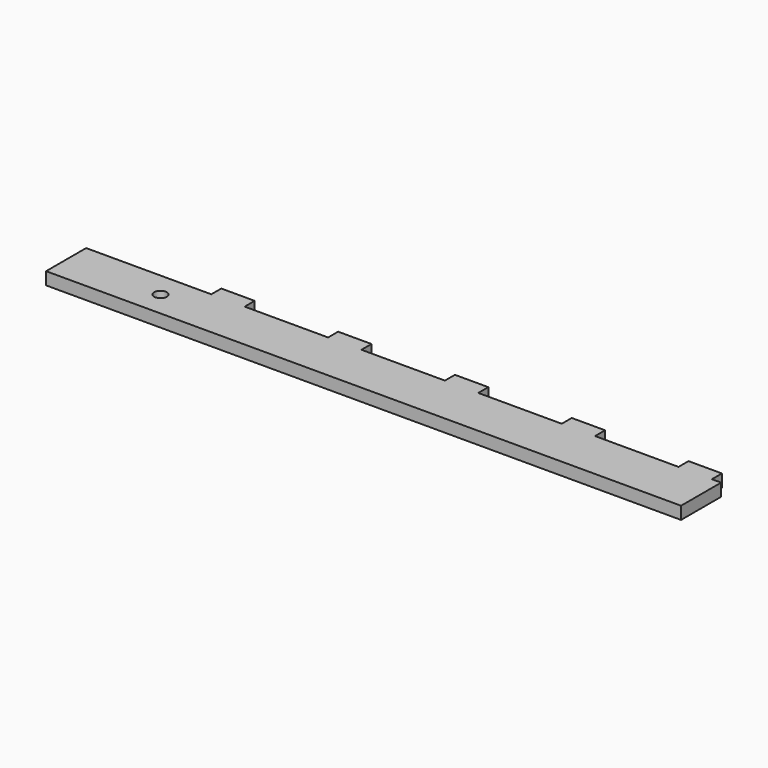
from build123d import *

# Parameters (mm, degrees)
F0_W     = 1143
F0_H     = 76.2
F1_DEPTH = 19.05
F2_W     = 50.8
F2_H     = 19.05
F3_DEPTH = 19.05
F4_R     = 9.525
F5_DEPTH = 19.05
F6_W     = 22.86
F6_H     = 15.875
F7_DEPTH = 25.4
F9_DEPTH = 25.4


# Not quite as in the source:
# - a length typed as a fraction of an inch, garbled in the dataset ("3 / 203.2 mm" for 3/8 in), is restored
# - a feature names something its author has since deleted; it is built from what else it names


with BuildPart() as f1:
    # F0 (on Top) → F1 (new body)
    with BuildSketch(Plane.XY):
        with Locations((571.5, -38.1)):
            Rectangle(F0_W, F0_H)
    extrude(amount=F1_DEPTH)

    # F2 (on face) → F3 (join)
    with BuildSketch(Plane(origin=(0, 0, 0), x_dir=(-1, 0, 0), z_dir=(0, 1, 0))):
        with Locations((-927.1, 9.525)):
            Rectangle(F2_W, F2_H)
        with Locations((-749.3, 9.525)):
            Rectangle(F2_W, F2_H)
        with Locations((-571.5, 9.525)):
            Rectangle(F2_W, F2_H)
        with Locations((-393.7, 9.525)):
            Rectangle(F2_W, F2_H)
        with Locations((-215.9, 9.525)):
            Rectangle(F2_W, F2_H)
    extrude(amount=F3_DEPTH)

    # F4 (on face) → F5 (cut)
    with BuildSketch(Plane.XY.offset(19.05)):
        with Locations((143.6968424, -38.1)):
            Circle(F4_R)
    extrude(amount=-F5_DEPTH, mode=Mode.SUBTRACT)

    # F6 (on face) → F7 (cut)
    with BuildSketch(Plane.XY.offset(19.05)):
        with Locations((1047.75, -7.9375)):
            Rectangle(F6_W, F6_H)
    extrude(amount=-F7_DEPTH, mode=Mode.SUBTRACT)

    # F8 (on face) → F9 (cut)
    with BuildSketch(Plane.XY.offset(19.05)):
        Polygon((1036.32, 0), (966.4863944054, 0), (966.4863944054, -76.2), (1143, -76.2), (1143, 0), (1059.18, 0), (1059.18, -15.875), (1036.32, -15.875), align=None)
    extrude(amount=-F9_DEPTH, mode=Mode.SUBTRACT)


solid = f1.part
